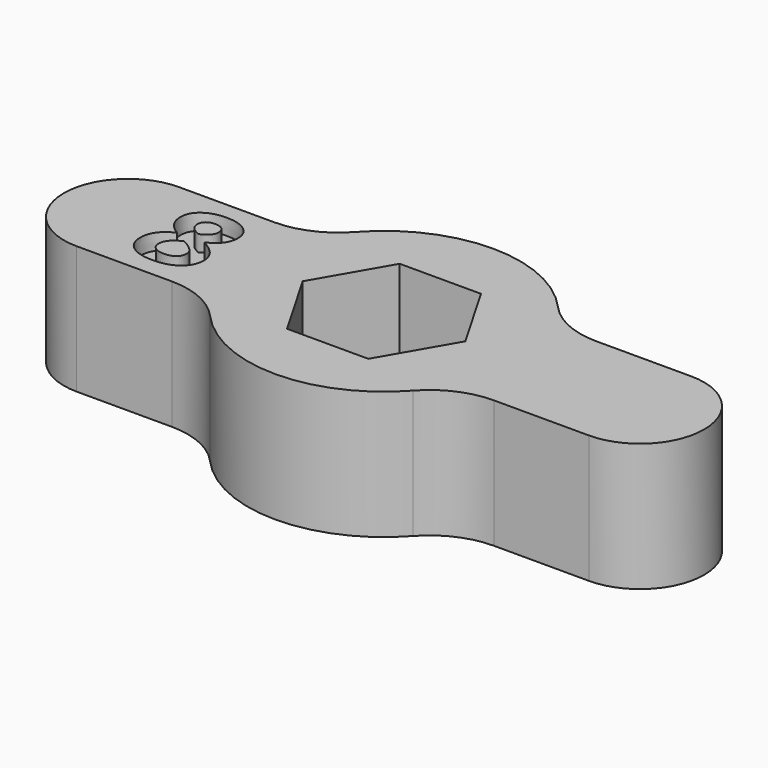
from build123d import *

# Parameters (mm, degrees)
F1_DEPTH     = 8
F2_TEXT_SIZE = 7.8653974924
F3_DEPTH     = 1
F4_R         = 5


# Not quite as in the source:
# - Text() gives the source's letters only with a copy of the font that has no kerning and outlines rounded to 1/6400 em; it was checked with that copy


with BuildPart() as f1:
    # F0 (on Top) → F1 (new body)
    with BuildSketch(Plane.XY):
        with BuildLine():
            ThreePointArc((-12.0228330124, -0.4579324492), (-13.0228330124, 3.5420675508), (-12.0228330124, 7.5420675508))
            Line((-12.0228330124, 7.5420675508), (-20.5228330124, 7.5420675508))
            ThreePointArc((-20.5228330124, 7.5420675508), (-24.5228330124, 3.5420675508), (-20.5228330124, -0.4579324492))
            Line((-20.5228330124, -0.4579324492), (-12.0228330124, -0.4579324492))
        make_face()
        with BuildLine():
            ThreePointArc((2.9771669876, -0.4579324492), (3.7233782388, 1.480514738), (3.9771669876, 3.5420675508))
            ThreePointArc((3.9771669876, 3.5420675508), (3.7233782388, 5.6036203636), (2.9771669876, 7.5420675508))
            ThreePointArc((2.9771669876, 7.5420675508), (-4.5228330124, 12.0420675508), (-12.0228330124, 7.5420675508))
            ThreePointArc((-12.0228330124, 7.5420675508), (-13.0228330124, 3.5420675508), (-12.0228330124, -0.4579324492))
            ThreePointArc((-12.0228330124, -0.4579324492), (-4.5228330124, -4.9579324492), (2.9771669876, -0.4579324492))
        make_face()
        Polygon((-1.982491828, 7.9420675508), (0.5578493565, 3.5420675508), (-1.982491828, -0.8579324492), (-7.0631741969, -0.8579324492), (-9.6035153813, 3.5420675508), (-7.0631741969, 7.9420675508), align=None, mode=Mode.SUBTRACT)
        with BuildLine():
            ThreePointArc((2.9771669876, 7.5420675508), (3.7233782388, 5.6036203636), (3.9771669876, 3.5420675508))
            ThreePointArc((3.9771669876, 3.5420675508), (3.7233782388, 1.480514738), (2.9771669876, -0.4579324492))
            Line((2.9771669876, -0.4579324492), (11.4771669876, -0.4579324492))
            ThreePointArc((11.4771669876, -0.4579324492), (15.4771669876, 3.5420675508), (11.4771669876, 7.5420675508))
            Line((11.4771669876, 7.5420675508), (2.9771669876, 7.5420675508))
        make_face()
    extrude(amount=F1_DEPTH)

    # F2 (on face) → F3 (cut)
    with BuildSketch(Plane.XY.offset(8)):
        with Locations((-18.9544288442, 0.7849140093)):
            Text('8', F2_TEXT_SIZE, font='Open Sans', font_style=FontStyle.BOLD, text_align=(TextAlign.LEFT, TextAlign.BOTTOM))
    extrude(amount=-F3_DEPTH, mode=Mode.SUBTRACT)

    # F4
    f4_edges = [f1.edges().sort_by_distance(p)[0] for p in [
        (2.977167, -0.457932, 4),
        (-12.022833, -0.457932, 4),
        (-12.022833, 7.542068, 4),
        (2.977167, 7.542068, 4),
    ]]
    fillet(f4_edges, radius=F4_R)


solid = f1.part
